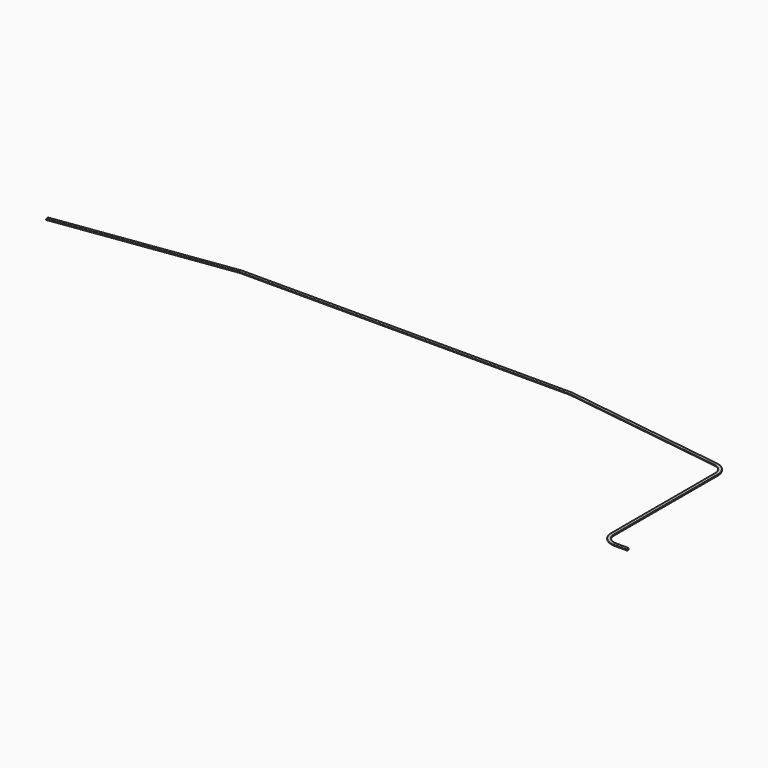
from build123d import *

# Parameters (mm, degrees)
F2_W = 24
F2_H = 12
F4_R = 5
F5_R = 11.99999


# Not quite as in the source:
# - a fillet or chamfer is up to 0.001 mm smaller than in the source, because OpenCascade refuses the exact size


with BuildPart() as f3:
    # F3: sweep along a path in F0
    with BuildLine(Plane.XY) as f3_path:
        Line((5642.5559538512, -1230), (5542.5559538512, -1230))
        ThreePointArc((5542.5559538512, -1230), (5471.8452757326, -1200.7106781187), (5442.5559538512, -1130))
        Line((5442.5559538512, -1130), (5442.5559538512, -86.9286737816))
        ThreePointArc((5442.5559538512, -86.9286737816), (5418.0269118735, -21.3227708826), (5356.4732639472, 12.0981330925))
        Line((5356.4732639472, 12.0981330925), (4053.2026058273, 195.2608792278))
        ThreePointArc((4053.2026058273, 195.2608792278), (4046.2609431057, 195.9904773797), (4039.2852957313, 196.2340723537))
        Line((4039.2852957313, 196.2340723537), (1403.27065812, 196.2340723537))
        ThreePointArc((1403.27065812, 196.2340723537), (1396.2950107456, 195.9904773797), (1389.353348024, 195.2608792278))
        Line((1389.353348024, 195.2608792278), (0, 0))
    # F2 (on line) → F3 (sweep)
    with BuildSketch(Plane.YZ.offset(5642.5559538512)):
        with Locations((-1230, -6)):
            Rectangle(F2_W, F2_H)
    sweep(path=f3_path.line)

    # F4
    f4_edges = [f3.edges().sort_by_distance(p)[0] for p in [
        (5592.555954, -1218, -12),
    ]]
    fillet(f4_edges, radius=F4_R)

    # F5 (radius 12 in the source; OpenCascade refuses exactly that, so slightly less here)
    f5_edges = [f3.edges().sort_by_distance(p)[0] for p in [
        (5592.555954, -1242, -12),
    ]]
    fillet(f5_edges, radius=F5_R)


solid = f3.part
